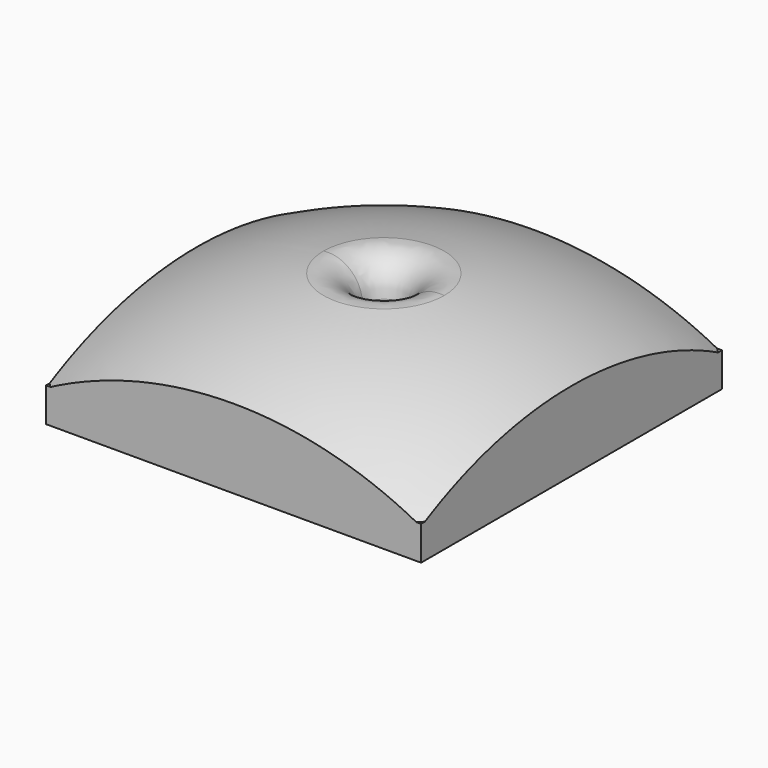
from build123d import *

# Parameters (mm, degrees)
F0_W     = 139.7
F0_H     = 139.7
F0_R     = 7.9375
F1_DEPTH = 12.7
F4_W     = 59.6992075443
F4_H     = 63.3541112766
F4_W_2   = 56.6389337182
F4_H_2   = 62.1770434082
F5_DEPTH = 101.6
F6_W     = 47.2303777933
F6_H     = 39.3290324137
F6_W_2   = 46.0887253284
F6_H_2   = 41.5412890725
F7_DEPTH = 101.6
F9_DEPTH = 76.2
F10_R    = 12.7


# Not quite as in the source:
# - a feature names something its author has since deleted; it is built from what else it names


with BuildPart() as f1:
    # F0 (on Top) → F1 (new body)
    with BuildSketch(Plane.XY):
        Rectangle(F0_W, F0_H)
        Circle(F0_R, mode=Mode.SUBTRACT)
    extrude(amount=F1_DEPTH)

    # F2 (on Front) → F3 (revolve)
    with BuildSketch(Plane.XZ):
        with BuildLine():
            Line((0, 0), (0, 45.1088836892))
            ThreePointArc((0, 45.1088836892), (-60.5414406288, 33.4106062222), (-112.3665997793, 0))
            Line((-112.3665997793, 0), (0, 0))
        make_face()
    revolve(axis=Axis((0, 0, 22.5544418446), (0, 0, -1)))

    # F4 (on Front) → F5 (cut, symmetric)
    with BuildSketch(Plane.XZ):
        with Locations((-99.4039475918, 19.7528828867)):
            Rectangle(F4_W, F4_H)
        with Locations((97.9946739972, 18.4055566788)):
            Rectangle(F4_W_2, F4_H_2)
    extrude(amount=F5_DEPTH, both=True, mode=Mode.SUBTRACT)

    # F6 (on Right) → F7 (cut, symmetric)
    with BuildSketch(Plane.YZ):
        with Locations((-93.4242233634, 10.9358266927)):
            Rectangle(F6_W, F6_H)
        with Locations((92.853397131, 9.8296983633)):
            Rectangle(F6_W_2, F6_H_2)
    extrude(amount=F7_DEPTH, both=True, mode=Mode.SUBTRACT)

    # F0 (on Top) → F9 (cut, symmetric)
    with BuildSketch(Plane.XY):
        Circle(F0_R)
    extrude(amount=F9_DEPTH, both=True, mode=Mode.SUBTRACT)

    # F10
    f10_edges = [f1.edges().sort_by_distance(p)[0] for p in [
        (0, -7.9375, 44.914919),
        (0, 7.9375, 44.914919),
    ]]
    fillet(f10_edges, radius=F10_R)


solid = f1.part
